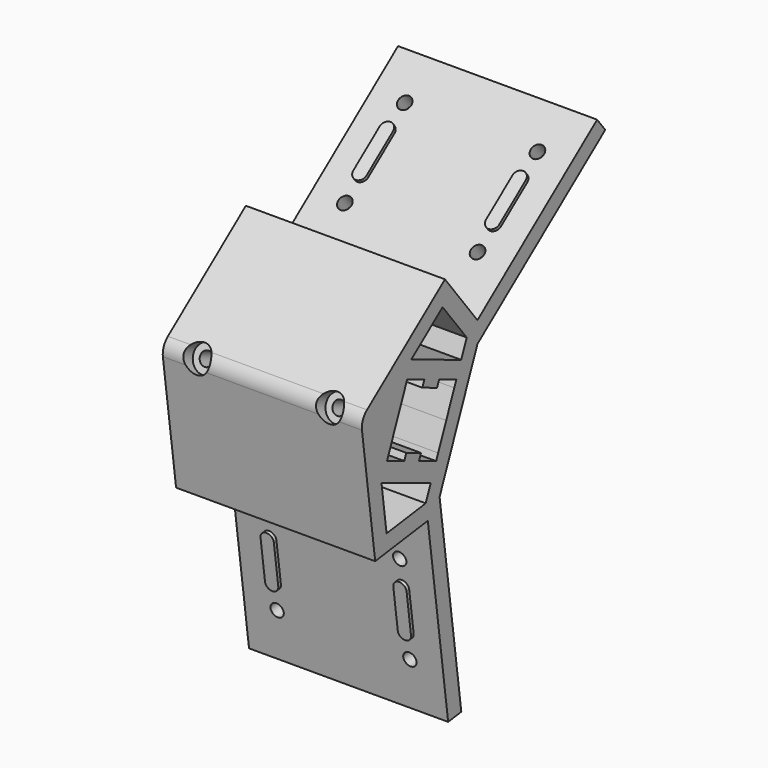
from build123d import *

# Parameters (mm, degrees)
F1_DEPTH  = 60
F2_DEPTH  = 5
F3_DEPTH  = 60
F4_R      = 5
F7_DEPTH  = 5
F8_DEPTH  = 5
F9_DEPTH  = 1
F10_DEPTH = 1
F12_DEPTH = 25
F13_DEPTH = 20
F14_DEPTH = 10


with BuildPart() as f1:
    # F0 (on Right) → F1 (new body)
    with BuildSketch(Plane.YZ):
        Polygon((-1.9545168432, 38.6489601963), (-33.5964987424, 14.1788767986), (-28.2257758369, -25.4589250511), (-8.406874912, -22.7735635983), (-0.7535947717, -79.2574312341), (4.2011304595, -78.5860908709), (-3.9713255886, -18.2705245759), (3.1545996335, -0.8816359607), (10.2805248557, 16.5072526545), (58.4291094867, 53.742590351), (55.370349062, 57.6978380884), (10.2805248557, 22.8279692467), align=None)
        Polygon((-25.8654488138, -5.6400241263), (-7.3142972833, -13.2422419285), (-9.1963342424, -17.8348428934), (-23.9423909688, -19.8328594567), align=None, mode=Mode.SUBTRACT)
        Polygon((1.5615552233, 8.4168698067), (-1.4719884671, 1.0143288458), (-4.5055321574, -6.3882121151), (-5.26391808, -8.2388473554), (-11.7411414209, -5.5844966263), (-17.2930471416, -3.3093388585), (-23.7702704824, -0.6549881294), (-23.0118845598, 1.1956471108), (-16.944797179, 16.0007290327), (-16.1864112564, 17.851364273), (-9.7091879156, 15.1970135439), (-4.1572821949, 12.9218557761), (2.3199411459, 10.267505047), align=None, mode=Mode.SUBTRACT)
        Polygon((-14.6534166938, 22.50764705), (-2.8510041559, 31.6349520341), (6.2523573083, 19.863500585), (4.1741345282, 14.7921613112), align=None, mode=Mode.SUBTRACT)
    extrude(amount=F1_DEPTH)

    # F0 (on Right) → F2 (join)
    with BuildSketch(Plane.YZ):
        Polygon((-16.944797179, 16.0007290327), (-10.4675738382, 13.3463783036), (-9.7091879156, 15.1970135439), (-16.1864112564, 17.851364273), align=None)
        Polygon((-4.9156681175, 11.0712205358), (1.5615552233, 8.4168698067), (2.3199411459, 10.267505047), (-4.1572821949, 12.9218557761), align=None)
        Polygon((-5.26391808, -8.2388473554), (-4.5055321574, -6.3882121151), (-10.9827554983, -3.7338613861), (-11.7411414209, -5.5844966263), align=None)
        Polygon((-17.2930471416, -3.3093388585), (-16.534661219, -1.4587036183), (-23.0118845598, 1.1956471108), (-23.7702704824, -0.6549881294), align=None)
    extrude(amount=F2_DEPTH)

    # F0 (on Right) → F3 (join)
    with BuildSketch(Plane.YZ):
        Polygon((-11.7411414209, -5.5844966263), (-10.9827554983, -3.7338613861), (-16.534661219, -1.4587036183), (-17.2930471416, -3.3093388585), align=None)
        Polygon((-10.4675738382, 13.3463783036), (-4.9156681175, 11.0712205358), (-4.1572821949, 12.9218557761), (-9.7091879156, 15.1970135439), align=None)
    extrude(amount=F3_DEPTH)

    # F4
    f4_edges = [f1.edges().sort_by_distance(p)[0] for p in [
        (30, -33.596499, 14.178877),
    ]]
    fillet(f4_edges, radius=F4_R)

    # F6 (on face) → F7 (cut)
    with BuildSketch(Plane(origin=(0, -11.2853910764, -1.5291137632), x_dir=(1, 0, 0), z_dir=(0, -0.9909450462, -0.1342680726))):
        with BuildLine():
            ThreePointArc((7.9984828914, -64.1860215089), (9.9984828914, -66.1860215089), (11.9984828914, -64.1860215089))
            ThreePointArc((11.9984828914, -64.1860215089), (9.9984828914, -62.1860215089), (7.9984828914, -64.1860215089))
        make_face()
        with BuildLine():
            ThreePointArc((7.9984828914, -35.6860233554), (9.9984828914, -37.6860233554), (11.9984828914, -35.6860233554))
            ThreePointArc((11.9984828914, -35.6860233554), (9.9984828914, -33.6860233554), (7.9984828914, -35.6860233554))
        make_face()
        with BuildLine():
            ThreePointArc((48.0015171086, -35.6972638628), (50.0015171086, -37.6972638628), (52.0015171086, -35.6972638628))
            ThreePointArc((52.0015171086, -35.6972638628), (50.0015171086, -33.6972638628), (48.0015171086, -35.6972638628))
        make_face()
        with BuildLine():
            ThreePointArc((48.0015171086, -64.1849918396), (50.0015171086, -66.1849918396), (52.0015171086, -64.1849918396))
            ThreePointArc((52.0015171086, -64.1849918396), (50.0015171086, -62.1849918396), (48.0015171086, -64.1849918396))
        make_face()
    extrude(amount=-F7_DEPTH, mode=Mode.SUBTRACT)

    # F5 (on face) → F8 (cut)
    with BuildSketch(Plane(origin=(0, -7.1996627103, 9.3098006026), x_dir=(1, 0, 0), z_dir=(0, -0.6117520849, 0.7910495475))):
        with BuildLine():
            ThreePointArc((48, 66.4655810893), (50, 64.4655810893), (52, 66.4655810893))
            ThreePointArc((52, 66.4655810893), (50, 68.4655810893), (48, 66.4655810893))
        make_face()
        with BuildLine():
            ThreePointArc((48, 37.9655810893), (50, 35.9655810893), (52, 37.9655810893))
            ThreePointArc((52, 37.9655810893), (50, 39.9655810893), (48, 37.9655810893))
        make_face()
        with BuildLine():
            ThreePointArc((8, 37.9655810893), (10, 35.9655810893), (12, 37.9655810893))
            ThreePointArc((12, 37.9655810893), (10, 39.9655810893), (8, 37.9655810893))
        make_face()
        with BuildLine():
            ThreePointArc((8, 66.4655810893), (10, 64.4655810893), (12, 66.4655810893))
            ThreePointArc((12, 66.4655810893), (10, 68.4655810893), (8, 66.4655810893))
        make_face()
    extrude(amount=-F8_DEPTH, mode=Mode.SUBTRACT)

    # F5 (on face) → F9 (join)
    with BuildSketch(Plane(origin=(0, -7.1996627103, 9.3098006026), x_dir=(1, 0, 0), z_dir=(0, -0.6117520849, 0.7910495475))):
        with BuildLine():
            ThreePointArc((48, 58.4655810893), (50, 56.4655810893), (52, 58.4655810893))
            ThreePointArc((52, 58.4655810893), (50, 60.4655810893), (48, 58.4655810893))
        make_face()
        with BuildLine():
            Line((52, 45.9655810893), (52, 58.4655810893))
            ThreePointArc((52, 58.4655810893), (50, 56.4655810893), (48, 58.4655810893))
            Line((48, 58.4655810893), (48, 45.9655810893))
            ThreePointArc((48, 45.9655810893), (50, 47.9655810893), (52, 45.9655810893))
        make_face()
        with BuildLine():
            ThreePointArc((48, 45.9655810893), (50, 43.9655810893), (52, 45.9655810893))
            ThreePointArc((52, 45.9655810893), (50, 47.9655810893), (48, 45.9655810893))
        make_face()
        with BuildLine():
            ThreePointArc((8, 58.4655810893), (10, 56.4655810893), (12, 58.4655810893))
            ThreePointArc((12, 58.4655810893), (10, 60.4655810893), (8, 58.4655810893))
        make_face()
        with BuildLine():
            ThreePointArc((8, 45.9655810893), (10, 47.9655810893), (12, 45.9655810893))
            Line((12, 45.9655810893), (12, 58.4655810893))
            ThreePointArc((12, 58.4655810893), (10, 56.4655810893), (8, 58.4655810893))
            Line((8, 58.4655810893), (8, 45.9655810893))
        make_face()
        with BuildLine():
            ThreePointArc((8, 45.9655810893), (10, 43.9655810893), (12, 45.9655810893))
            ThreePointArc((12, 45.9655810893), (10, 47.9655810893), (8, 45.9655810893))
        make_face()
    extrude(amount=F9_DEPTH)

    # F6 (on face) → F10 (join)
    with BuildSketch(Plane(origin=(0, -11.2853910764, -1.5291137632), x_dir=(1, 0, 0), z_dir=(0, -0.9909450462, -0.1342680726))):
        with BuildLine():
            ThreePointArc((48.0015171086, -43.6972638628), (50.0015171086, -45.6972638628), (52.0015171086, -43.6972638628))
            ThreePointArc((52.0015171086, -43.6972638628), (50.0015171086, -41.6972638628), (48.0015171086, -43.6972638628))
        make_face()
        with BuildLine():
            Line((52.0015171086, -56.1849918396), (52.0015171086, -43.6972638628))
            ThreePointArc((52.0015171086, -43.6972638628), (50.0015171086, -45.6972638628), (48.0015171086, -43.6972638628))
            Line((48.0015171086, -43.6972638628), (48.0015171086, -56.1849918396))
            ThreePointArc((48.0015171086, -56.1849918396), (50.0015171086, -54.1849918396), (52.0015171086, -56.1849918396))
        make_face()
        with BuildLine():
            ThreePointArc((48.0015171086, -56.1849918396), (50.0015171086, -58.1849918396), (52.0015171086, -56.1849918396))
            ThreePointArc((52.0015171086, -56.1849918396), (50.0015171086, -54.1849918396), (48.0015171086, -56.1849918396))
        make_face()
        with BuildLine():
            ThreePointArc((7.9984828914, -43.6860233554), (9.9984828914, -45.6860233554), (11.9984828914, -43.6860233554))
            ThreePointArc((11.9984828914, -43.6860233554), (9.9984828914, -41.6860233554), (7.9984828914, -43.6860233554))
        make_face()
        with BuildLine():
            ThreePointArc((7.9984828914, -56.1860215089), (9.9984828914, -54.1860215089), (11.9984828914, -56.1860215089))
            Line((11.9984828914, -56.1860215089), (11.9984828914, -43.6860233554))
            ThreePointArc((11.9984828914, -43.6860233554), (9.9984828914, -45.6860233554), (7.9984828914, -43.6860233554))
            Line((7.9984828914, -43.6860233554), (7.9984828914, -56.1860215089))
        make_face()
        with BuildLine():
            ThreePointArc((7.9984828914, -56.1860215089), (9.9984828914, -58.1860215089), (11.9984828914, -56.1860215089))
            ThreePointArc((11.9984828914, -56.1860215089), (9.9984828914, -54.1860215089), (7.9984828914, -56.1860215089))
        make_face()
    extrude(amount=F10_DEPTH)

    # F11 (on face) → F12 (cut)
    with BuildSketch(Plane(origin=(0, -20.1225891662, 8.2461892101), x_dir=(-1, 0, 0), z_dir=(0, 0.9253176201, -0.3791929613))):
        with BuildLine():
            Line((-12, 0.3804086878), (-8, 0.3804086878))
            ThreePointArc((-8, 0.3804086878), (-10, 2.3804086878), (-12, 0.3804086878))
        make_face()
        with BuildLine():
            Line((-52, 0.3804086878), (-48, 0.3804086878))
            ThreePointArc((-48, 0.3804086878), (-50, 2.3804086878), (-52, 0.3804086878))
        make_face()
        with BuildLine():
            ThreePointArc((-52, 0.3804086878), (-50, -1.6195913122), (-48, 0.3804086878))
            Line((-48, 0.3804086878), (-52, 0.3804086878))
        make_face()
        with BuildLine():
            ThreePointArc((-12, 0.3804086878), (-10, -1.6195913122), (-8, 0.3804086878))
            Line((-8, 0.3804086878), (-12, 0.3804086878))
        make_face()
    extrude(amount=-F12_DEPTH, mode=Mode.SUBTRACT)

    # F11 (on face) → F13 (join)
    with BuildSketch(Plane(origin=(0, -20.1225891662, 8.2461892101), x_dir=(-1, 0, 0), z_dir=(0, 0.9253176201, -0.3791929613))):
        with BuildLine():
            Line((-48, 0.3804086878), (-46, 0.3804086878))
            ThreePointArc((-46, 0.3804086878), (-50, 4.3804086878), (-54, 0.3804086878))
            Line((-54, 0.3804086878), (-52, 0.3804086878))
            ThreePointArc((-52, 0.3804086878), (-50, 2.3804086878), (-48, 0.3804086878))
        make_face()
        with BuildLine():
            ThreePointArc((-54, 0.3804086878), (-50, -3.6195913122), (-46, 0.3804086878))
            Line((-46, 0.3804086878), (-48, 0.3804086878))
            ThreePointArc((-48, 0.3804086878), (-50, -1.6195913122), (-52, 0.3804086878))
            Line((-52, 0.3804086878), (-54, 0.3804086878))
        make_face()
        with BuildLine():
            ThreePointArc((-14, 0.3804086878), (-10, -3.6195913122), (-6, 0.3804086878))
            Line((-6, 0.3804086878), (-8, 0.3804086878))
            ThreePointArc((-8, 0.3804086878), (-10, -1.6195913122), (-12, 0.3804086878))
            Line((-12, 0.3804086878), (-14, 0.3804086878))
        make_face()
        with BuildLine():
            Line((-8, 0.3804086878), (-6, 0.3804086878))
            ThreePointArc((-6, 0.3804086878), (-10, 4.3804086878), (-14, 0.3804086878))
            Line((-14, 0.3804086878), (-12, 0.3804086878))
            ThreePointArc((-12, 0.3804086878), (-10, 2.3804086878), (-8, 0.3804086878))
        make_face()
    extrude(amount=-F13_DEPTH)

    # F14 (cut): faces of the model
    f14_faces = [f1.faces().sort_by_distance(p)[0] for p in [
        (7.886862915, -38.4846932718, 16.1820472977),
        (46.113137085, -38.4846932718, 16.1820472977),
    ]]
    extrude(f14_faces, amount=-F14_DEPTH, mode=Mode.SUBTRACT)


solid = f1.part
